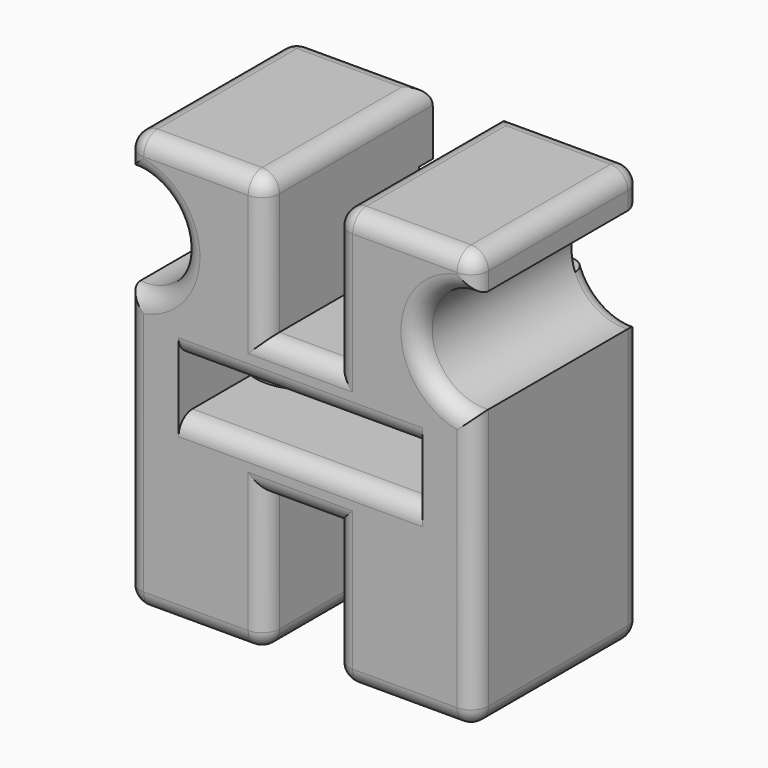
from build123d import *

# Parameters (mm, degrees)
F1_DEPTH = 60
F2_W     = 70
F2_H     = 15
F3_DEPTH = 50
F4_R     = 15
F5_R     = 15
F6_DEPTH = 67.5
F7_W     = 20
F7_H     = 12
F8_DEPTH = 5
F9_R     = 4.99999


# Not quite as in the source:
# - a fillet or chamfer is up to 0.001 mm smaller than in the source, because OpenCascade refuses the exact size


with BuildPart() as f1:
    # F0 (on Front) → F1 (new body)
    with BuildSketch(Plane.XZ):
        with BuildLine():
            Line((-8.0390890029, 59.2476050396), (-48.0390890029, 59.2476050396))
            Line((-48.0390890029, 59.2476050396), (-48.0390890029, 49.1578779955))
            ThreePointArc((-48.0390890029, 49.1578779955), (-31.8798250439, 34.2027415175), (-48.0390890029, 19.2476050396))
            Line((-48.0390890029, 19.2476050396), (-48.0390890029, -60.7523949604))
            Line((-48.0390890029, -60.7523949604), (-8.0390890029, -60.7523949604))
            Line((-8.0390890029, -60.7523949604), (-8.0390890029, -20.7523949604))
            Line((-8.0390890029, -20.7523949604), (11.9609109971, -20.7523949604))
            Line((11.9609109971, -20.7523949604), (11.9609109971, -60.7523949604))
            Line((11.9609109971, -60.7523949604), (51.9609109971, -60.7523949604))
            Line((51.9609109971, -60.7523949604), (51.9609109971, 19.2476050396))
            ThreePointArc((51.9609109971, 19.2476050396), (35.8016470382, 34.2027415175), (51.9609109971, 49.1578779955))
            Line((51.9609109971, 49.1578779955), (51.9609109971, 59.2476050396))
            Line((51.9609109971, 59.2476050396), (11.9609109971, 59.2476050396))
            Line((11.9609109971, 59.2476050396), (11.9609109971, 19.2476050396))
            Line((11.9609109971, 19.2476050396), (-8.0390890029, 19.2476050396))
            Line((-8.0390890029, 19.2476050396), (-8.0390890029, 59.2476050396))
        make_face()
    extrude(amount=F1_DEPTH)

    # F2 (on face) → F3 (cut)
    with BuildSketch(Plane.XZ.offset(60)):
        with Locations((1.9609109971, -0.7523949604)):
            Rectangle(F2_W, F2_H)
    extrude(amount=-F3_DEPTH, mode=Mode.SUBTRACT)

    # F4 (on face) + F5 (on face) → F6 (cut)
    with BuildSketch(Plane(origin=(0, 0, -60.7523949604), x_dir=(1, 0, 0), z_dir=(0, 0, -1))):
        with Locations((-28.0390890029, 20)):
            Circle(F4_R)
    with BuildSketch(Plane(origin=(0, 0, -60.7523949604), x_dir=(1, 0, 0), z_dir=(0, 0, -1))):
        with Locations((31.9609109971, 20)):
            Circle(F5_R)
    extrude(amount=-F6_DEPTH, mode=Mode.SUBTRACT)

    # F7 (on face) → F8 (cut)
    with BuildSketch(Plane.XZ):
        with BuildLine():
            Line((37.9935329711, 28.6991419792), (37.9935329711, 40.6991419792))
            Line((37.9935329711, 40.6991419792), (37.281411055, 40.6991419792))
            ThreePointArc((37.281411055, 40.6991419792), (35.811430972, 34.7444261941), (36.8477804729, 28.6991419792))
            Line((36.8477804729, 28.6991419792), (37.9935329711, 28.6991419792))
        make_face()
        with Locations((1.9609109971, 34.6991419792)):
            Rectangle(F7_W, F7_H)
        with BuildLine():
            Line((-8.0390890029, 28.6991419792), (-8.0390890029, 40.6991419792))
            Line((-8.0390890029, 40.6991419792), (-33.3595890607, 40.6991419792))
            ThreePointArc((-33.3595890607, 40.6991419792), (-31.8896089777, 34.7444261941), (-32.9259584786, 28.6991419792))
            Line((-32.9259584786, 28.6991419792), (-8.0390890029, 28.6991419792))
        make_face()
        with BuildLine():
            ThreePointArc((-32.9259584786, 28.6991419792), (-31.8896089777, 34.7444261941), (-33.3595890607, 40.6991419792))
            Line((-33.3595890607, 40.6991419792), (-38.3973060106, 40.6991419792))
            Line((-38.3973060106, 40.6991419792), (-38.3973060106, 28.6991419792))
            Line((-38.3973060106, 28.6991419792), (-32.9259584786, 28.6991419792))
        make_face()
        with BuildLine():
            ThreePointArc((36.8477804729, 28.6991419792), (35.811430972, 34.7444261941), (37.281411055, 40.6991419792))
            Line((37.281411055, 40.6991419792), (11.9609109971, 40.6991419792))
            Line((11.9609109971, 40.6991419792), (11.9609109971, 28.6991419792))
            Line((11.9609109971, 28.6991419792), (36.8477804729, 28.6991419792))
        make_face()
    extrude(amount=F8_DEPTH, mode=Mode.SUBTRACT)

    # F9 (radius 5 in the source; OpenCascade refuses exactly that, so slightly less here)
    f9_edges = [f1.edges().sort_by_distance(p)[0] for p in [
        (-31.879825, -60, 34.202742),
        (-48.039089, -60, 54.202742),
        (-28.039089, -60, 59.247605),
        (-8.039089, -60, 39.247605),
        (1.960911, -60, 19.247605),
        (11.960911, -60, 39.247605),
        (31.960911, -60, 59.247605),
        (51.960911, -60, 54.202742),
        (35.801647, -60, 34.202742),
        (51.960911, -60, -20.752395),
        (-48.039089, -60, -20.752395),
        (-28.039089, -60, -60.752395),
        (31.960911, -60, -60.752395),
        (11.960911, -60, -40.752395),
        (-8.039089, -60, -40.752395),
        (1.960911, -60, -20.752395),
        (1.960911, -60, -8.252395),
        (1.960911, -60, 6.747605),
        (51.960911, -30, 59.247605),
        (11.960911, -30, 59.247605),
        (-8.039089, -30, 59.247605),
        (-48.039089, -30, 59.247605),
        (31.960911, 0, 59.247605),
        (-28.039089, 0, 59.247605),
        (43.312591, 0, 47.199435),
        (42.848135, 0, 21.484973),
        (-38.926313, 0, 21.484973),
        (-39.390769, 0, 47.199435),
        (51.960911, 0, 54.202742),
        (-48.039089, 0, 54.202742),
        (-48.039089, 0, -20.752395),
        (51.960911, 0, -20.752395),
        (-28.039089, 0, -60.752395),
        (31.960911, 0, -60.752395),
        (-8.039089, 0, -40.752395),
        (11.960911, 0, -40.752395),
        (1.960911, 0, -20.752395),
        (11.960911, -30, -60.752395),
        (-8.039089, -30, -60.752395),
        (-48.039089, -30, -60.752395),
        (51.960911, -30, -60.752395),
    ]]
    fillet(f9_edges, radius=F9_R)


solid = f1.part
